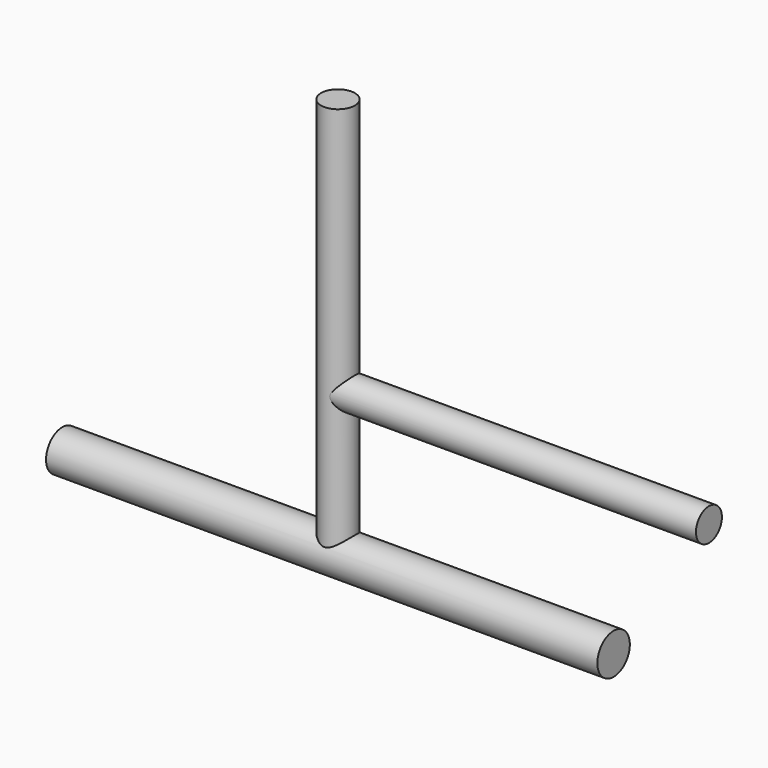
from build123d import *

# Parameters (mm, degrees)
F0_R          = 23.1250603282
F1_DEPTH      = 711.2
F2_R          = 44.8716829259
F3_DEPTH      = 609.6
F3_DEPTH_BACK = 609.6
F4_R          = 37.4216193061
F5_DEPTH      = 881.38
F8_R          = 35.8974591154
F9_DEPTH      = 820.42


# Not quite as in the source:
# - a feature of the source that left no trace in its solid (it failed there, or was rolled back) is left out


with BuildPart() as f1:
    # F0 (on Top) → F1 (new body)
    with BuildSketch(Plane.XY):
        Circle(F0_R)
    extrude(amount=F1_DEPTH)

    # F2 (on Right) → F3 (join, two sides)
    with BuildSketch(Plane.YZ) as f3_sk:
        Circle(F2_R)
    extrude(amount=F3_DEPTH)
    extrude(f3_sk.sketch, amount=-F3_DEPTH_BACK)

    # F4 (on Top) → F5 (join)
    with BuildSketch(Plane.XY):
        Circle(F4_R)
    extrude(amount=F5_DEPTH)

    # F8 (on Right) → F9 (join)
    with BuildSketch(Plane.YZ):
        with Locations((0, 320.2763795853)):
            Circle(F8_R)
    extrude(amount=F9_DEPTH)


solid = f1.part
